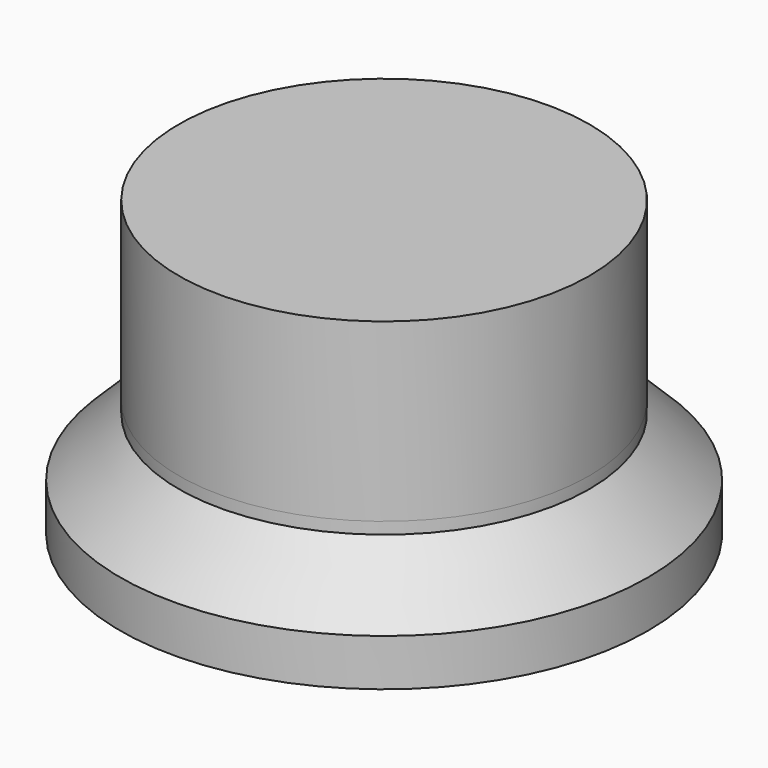
from build123d import *

# Parameters (mm, degrees)
F0_R        = 22.5
F0_R_2      = 17.5
F1_DEPTH    = 10
F2_DEPTH    = 25
F3_S5_R     = 17.5
F3_T6_DEPTH = 33


# Not quite as in the source:
# - a fillet or chamfer that OpenCascade refuses, or shapes differently, is made with other operations: its cross-section is extruded or revolved along the edge and cut away or added


with BuildPart() as f1:
    # F0 (on Top) → F1 (new body)
    with BuildSketch(Plane.XY):
        Circle(F0_R)
        Circle(F0_R_2, mode=Mode.SUBTRACT)
    extrude(amount=F1_DEPTH)

    # F0 (on Top) → F2 (join)
    with BuildSketch(Plane.XY):
        Circle(F0_R_2)
    extrude(amount=F2_DEPTH)

    # F3: chamfer of 6 on 1 edges, made by hand


with BuildPart() as f3_tool2:
    # F3_s3 → F3_t4 (revolve)
    with BuildSketch(Plane.XZ):
        Polygon((22.5, 4), (16.5, 10), (22.5, 10), align=None)
    revolve(axis=Axis((0, 0, 10), (0, 0, 1)))

    # F3_s5 → F3_t6 (cut, symmetric)
    with BuildSketch(Plane.XY.offset(7)):
        Circle(F3_S5_R)
    extrude(amount=F3_T6_DEPTH, both=True, mode=Mode.SUBTRACT)


with BuildPart() as f1_1:
    add(f1.part)

    # F3_t1: cut F3_tool2
    add(f3_tool2.part, mode=Mode.SUBTRACT)


solid = f1_1.part
